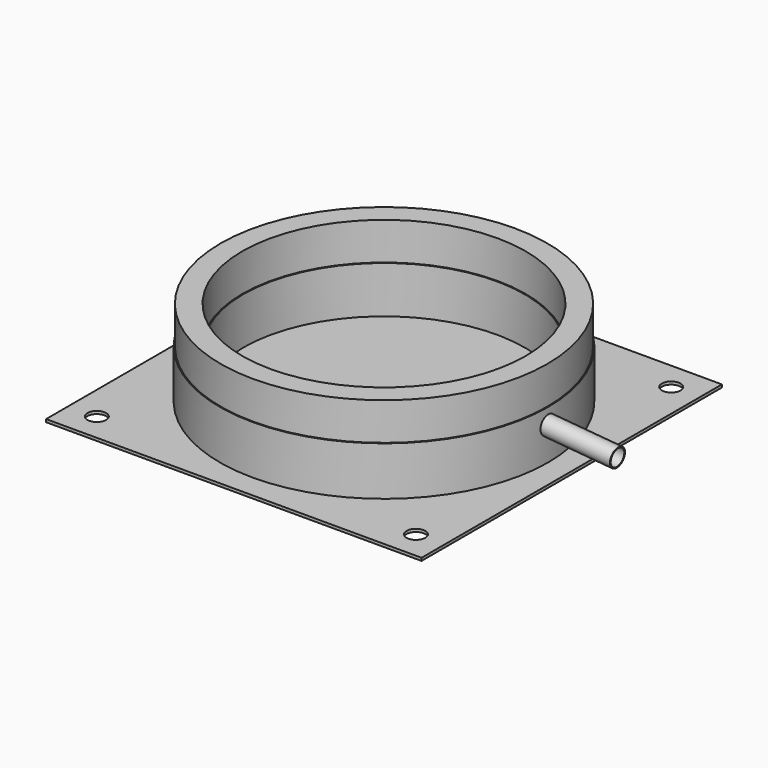
from build123d import *

# Parameters (mm, degrees)
F0_W     = 10
F0_H     = 3
F2_W     = 400
F2_H     = 400
F2_R     = 10
F3_DEPTH = 3
F6_R     = 9
F7_DEPTH = 120
F8_R     = 150
F9_DEPTH = 200


with BuildPart() as f1:
    # F0 (on Front) → F1 (revolve)
    with BuildSketch(Plane.XZ):
        Polygon((-175, 5), (-150, 5), (-150, 55), (-151, 55), (-151, 95), (-174, 95), (-174, 55), (-175, 55), align=None)
        Polygon((-10, 5), (-150, 5), (-175, 5), (-175, 2), (-10, 2), align=None)
        with Locations((-5, 3.5)):
            Rectangle(F0_W, F0_H)
    revolve(axis=Axis((0, 0, 187.9212413023), (0, 0, -1)))

    # F2 (on Top) → F3 (join)
    with BuildSketch(Plane.XY):
        Rectangle(F2_W, F2_H)
        with Locations((-170, -170)):
            Circle(F2_R, mode=Mode.SUBTRACT)
        with Locations((170, -170)):
            Circle(F2_R, mode=Mode.SUBTRACT)
        with Locations((-170, 170)):
            Circle(F2_R, mode=Mode.SUBTRACT)
        with Locations((170, 170)):
            Circle(F2_R, mode=Mode.SUBTRACT)
    extrude(amount=F3_DEPTH)

    # F4 (on Front) → F5 (revolve)
    with BuildSketch(Plane.XZ):
        Polygon((249.6194698092, 41.5098406888), (150, 50.2254149636), (149.9128442573, 49.2292202655), (249.5323140664, 40.5136459907), align=None)
    revolve(axis=Axis((262.7442754949, 0, 30.3233706049), (0.9961946981, 0, -0.0871557427)))

    # F6 (on face) → F7 (cut)
    with BuildSketch(Plane(origin=(244.1192753946, 0, -21.3576691452), x_dir=(0, 1, 0), z_dir=(0.9961946981, 0, -0.0871557427))):
        with Locations((0, 53.1076535083)):
            Circle(F6_R)
    extrude(amount=-F7_DEPTH, mode=Mode.SUBTRACT)

    # F8 (on face) → F9 (cut)
    with BuildSketch(Plane.XY.offset(5)):
        Circle(F8_R)
    extrude(amount=F9_DEPTH, mode=Mode.SUBTRACT)


solid = f1.part
